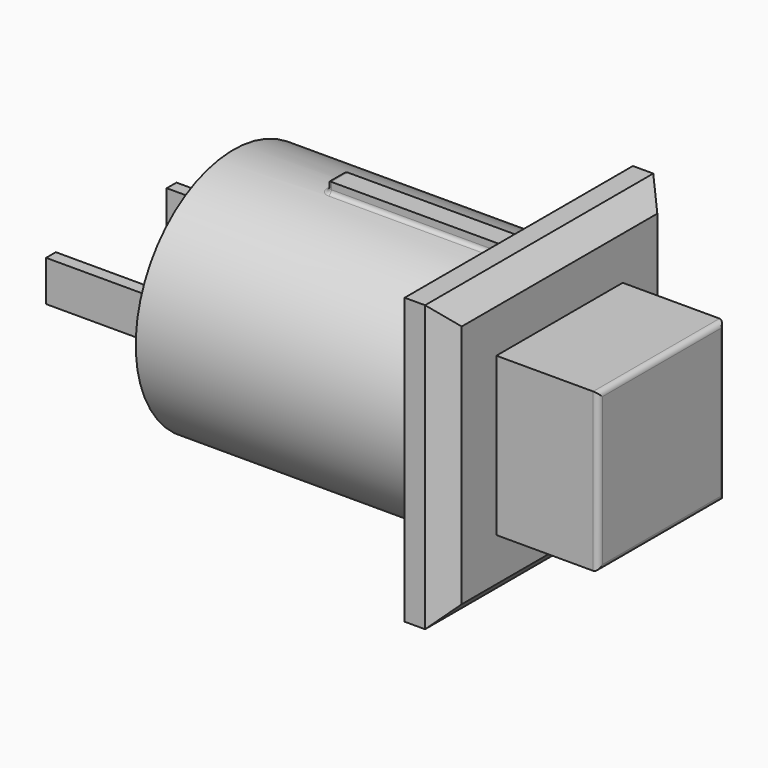
from build123d import *

# Parameters (mm, degrees)
F0_R      = 6
F1_DEPTH  = 14
F2_W      = 14
F2_H      = 14
F3_DEPTH  = 2
F4_W      = 7.75
F4_H      = 7.75
F5_DEPTH  = 5
F6_W      = 0.6
F6_H      = 2
F7_DEPTH  = 6
F8_R      = 0.25
F9_SIZE   = 1
F11_DEPTH = 9
F12_R     = 0.2


with BuildPart() as f1:
    # F0 (on Right) → F1 (new body)
    with BuildSketch(Plane.YZ):
        Circle(F0_R)
    extrude(amount=F1_DEPTH)

    # F2 (on face) → F3 (join)
    with BuildSketch(Plane.YZ.offset(14)):
        Rectangle(F2_W, F2_H)
    extrude(amount=F3_DEPTH)

    # F4 (on face) → F5 (join)
    with BuildSketch(Plane.YZ.offset(16)):
        Rectangle(F4_W, F4_H)
    extrude(amount=F5_DEPTH)

    # F6 (on face) → F7 (join)
    with BuildSketch(Plane(origin=(0, 0, 0), x_dir=(0, -1, 0), z_dir=(-1, 0, 0))):
        with Locations((-3.7, 0)):
            Rectangle(F6_W, F6_H)
        with Locations((3.7, 0)):
            Rectangle(F6_W, F6_H)
    extrude(amount=F7_DEPTH)

    # F8
    f8_edges = [f1.edges().sort_by_distance(p)[0] for p in [
        (21, 0, 3.875),
        (21, -3.875, 0),
        (21, 0, -3.875),
        (21, 3.875, 0),
    ]]
    fillet(f8_edges, radius=F8_R)

    # F9
    f9_edges = [f1.edges().sort_by_distance(p)[0] for p in [
        (16, 0, -7),
        (16, -7, 0),
        (16, 0, 7),
        (16, 7, 0),
    ]]
    chamfer(f9_edges, length=F9_SIZE)

    # F10 (on face) → F11 (join)
    with BuildSketch(Plane(origin=(14, 0, 0), x_dir=(0, -1, 0), z_dir=(-1, 0, 0))):
        Polygon((0.5, 6.5), (-0.5, 6.5), (-0.5, 6), (-0.5, 5.9002675116), (0.5, 5.9002675116), (0.5, 6), align=None)
    extrude(amount=F11_DEPTH)

    # F12
    f12_edges = [f1.edges().sort_by_distance(p)[0] for p in [
        (5, -0.5, 6.239565),
        (5, 0, 6),
        (5, 0.5, 6.239565),
        (5, 0, 6.5),
        (9.5, -0.5, 5.97913),
        (9.5, 0.5, 5.97913),
    ]]
    fillet(f12_edges, radius=F12_R)


solid = f1.part
